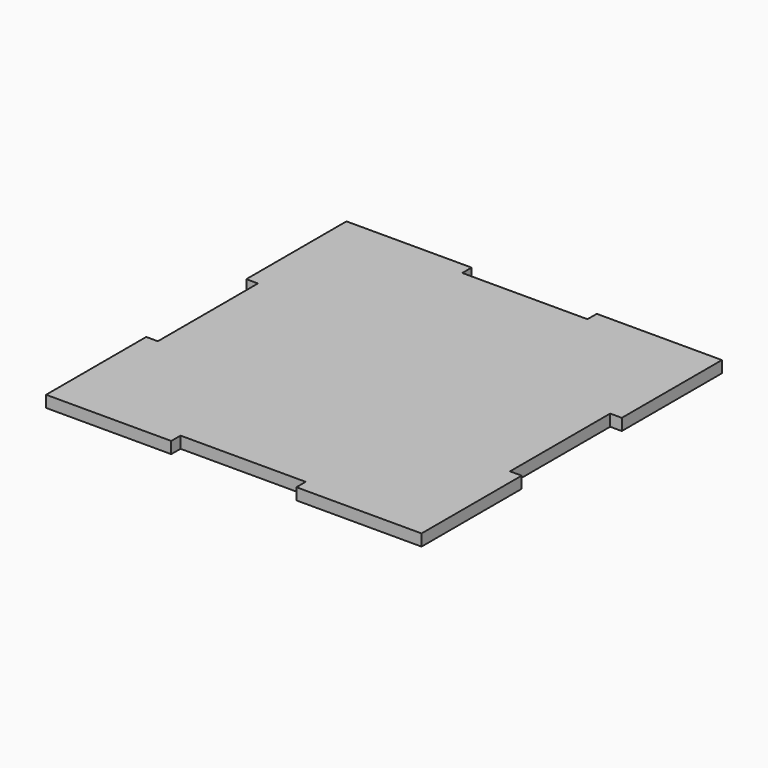
from build123d import *

# Parameters (mm, degrees)
F0_W            = 76.2
F0_H            = 76.2
F1_DEPTH        = 2.3622
F2_W            = 25.4
F2_H            = 2.3622
F4_DEPTH        = 25.4
F4_COPIES_COUNT = 4


# Not quite as in the source:
# - a pattern or mirror of a feature is missing from the dataset's text; its kind, count and spacing are read off the source's solid


with BuildPart() as f1:
    # F0 (on Top) → F1 (new body)
    with BuildSketch(Plane.XY):
        Rectangle(F0_W, F0_H)
    extrude(amount=F1_DEPTH)

    # F2 (on face) → F4 (cut)
    with BuildSketch(Plane.XY.offset(2.3622)):
        with Locations((0, 36.9189)):
            Rectangle(F2_W, F2_H)
    f4 = extrude(amount=-F4_DEPTH, mode=Mode.SUBTRACT)

    # F4_copies: F4 ×4 about axis
    f4_copies_axis = Axis((0, 0, 0), (0, 0, 1))
    for i in range(1, F4_COPIES_COUNT):
        add(f4.rotate(f4_copies_axis, i * 360 / F4_COPIES_COUNT), mode=Mode.SUBTRACT)


solid = f1.part
